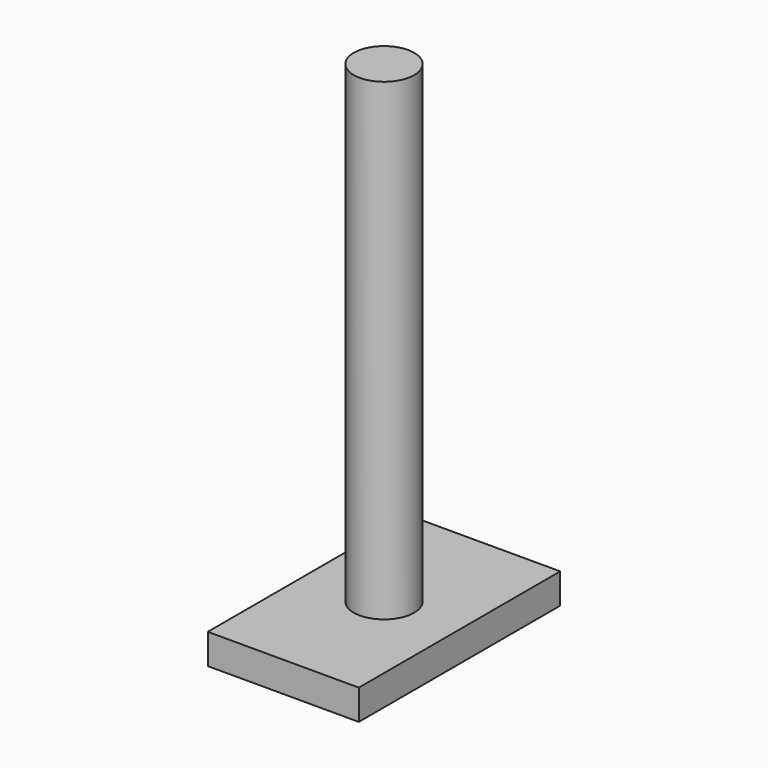
from build123d import *

# Parameters (mm, degrees)
F0_W     = 15
F0_H     = 25
F1_DEPTH = 3
F2_R     = 3
F3_DEPTH = 50


# Not quite as in the source:
# - a feature names something its author has since deleted; it is built from what else it names


with BuildPart() as f1:
    # F0 (on Top) → F1 (new body)
    with BuildSketch(Plane.XY):
        Rectangle(F0_W, F0_H)
    extrude(amount=F1_DEPTH)

    # F2 (on Top) → F3 (join)
    with BuildSketch(Plane.XY):
        Circle(F2_R)
    extrude(amount=F3_DEPTH)


solid = f1.part
